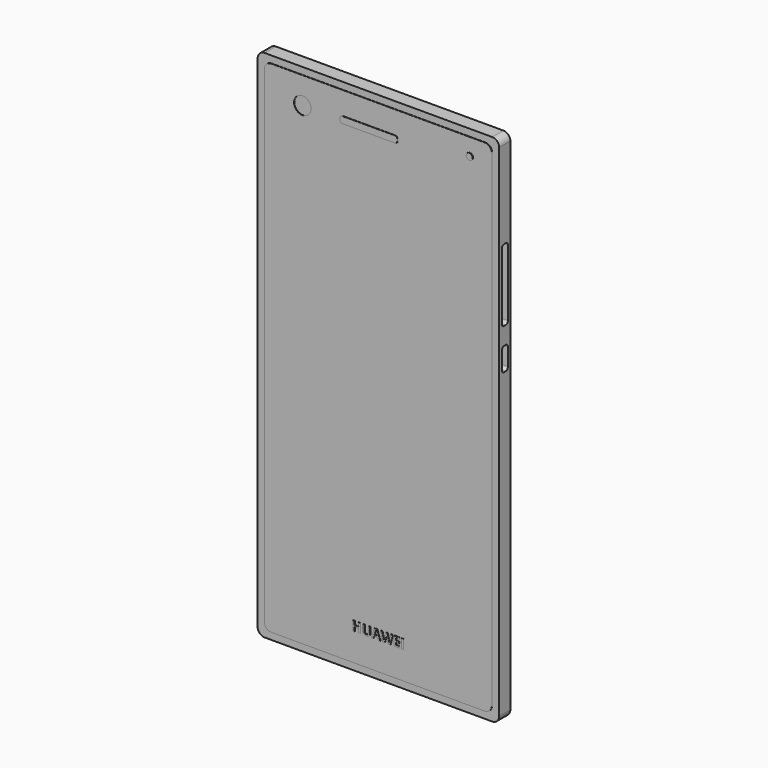
from build123d import *

# Parameters (mm, degrees)
F1_DEPTH      = 4
F3_DEPTH      = 2
F5_DEPTH      = 0.1
F6_W          = 64.8
F6_H          = 111
F7_DEPTH      = 0.1
F9_DEPTH      = 0.1
F10_R         = 2.4467451842
F11_DEPTH     = 0.1
F12_R         = 0.9273292915
F13_DEPTH     = 0.1
F14_TEXT_SIZE = 3.7091414883
F15_DEPTH     = 0.1


# Not quite as in the source:
# - Text() gives the source's letters only with a copy of the font that has no kerning and outlines rounded to 1/6400 em; it was checked with that copy


with BuildPart() as f1:
    # F0 (on Front) → F1 (new body)
    with BuildSketch(Plane.XZ):
        with BuildLine():
            ThreePointArc((-2, 0), (-0.5857864376, 0.5857864376), (0, 2))
            Line((0, 2), (0, 145))
            ThreePointArc((0, 145), (-0.5857864376, 146.4142135624), (-2, 147))
            Line((-2, 147), (-67, 147))
            ThreePointArc((-67, 147), (-68.4142135624, 146.4142135624), (-69, 145))
            Line((-69, 145), (-69, 2))
            ThreePointArc((-69, 2), (-68.4142135624, 0.5857864376), (-67, 0))
            Line((-67, 0), (-2, 0))
        make_face()
    extrude(amount=F1_DEPTH)

    # F2 (on face) → F3 (cut)
    with BuildSketch(Plane.YZ):
        with BuildLine():
            Line((-1.6547506675, 120), (-2.2547506675, 120))
            ThreePointArc((-2.2547506675, 120), (-2.8204360925, 119.7656854249), (-3.0547506675, 119.2))
            Line((-3.0547506675, 119.2), (-3.0547506675, 100.2))
            ThreePointArc((-3.0547506675, 100.2), (-2.8204360925, 99.6343145751), (-2.2547506675, 99.4))
            Line((-2.2547506675, 99.4), (-1.6547506675, 99.4))
            ThreePointArc((-1.6547506675, 99.4), (-1.0890652426, 99.6343145751), (-0.8547506675, 100.2))
            Line((-0.8547506675, 100.2), (-0.8547506675, 119.2))
            ThreePointArc((-0.8547506675, 119.2), (-1.0890652426, 119.7656854249), (-1.6547506675, 120))
        make_face()
        with BuildLine():
            Line((-1.6547506675, 94.4), (-2.2547506675, 94.4))
            ThreePointArc((-2.2547506675, 94.4), (-2.8204360925, 94.1656854249), (-3.0547506675, 93.6))
            Line((-3.0547506675, 93.6), (-3.0547506675, 88.6))
            ThreePointArc((-3.0547506675, 88.6), (-2.8204360925, 88.0343145751), (-2.2547506675, 87.8))
            Line((-2.2547506675, 87.8), (-1.6547506675, 87.8))
            ThreePointArc((-1.6547506675, 87.8), (-1.0890652426, 88.0343145751), (-0.8547506675, 88.6))
            Line((-0.8547506675, 88.6), (-0.8547506675, 93.6))
            ThreePointArc((-0.8547506675, 93.6), (-1.0890652426, 94.1656854249), (-1.6547506675, 94.4))
        make_face()
    extrude(amount=-F3_DEPTH, mode=Mode.SUBTRACT)

    # F6 (on face) → F7 (join)
    with BuildSketch(Plane.XZ.offset(4)):
        with Locations((-34.5, 75.5)):
            Rectangle(F6_W, F6_H)
    extrude(amount=F7_DEPTH)


with BuildPart() as f5:
    # F4 (on face) → F5 (new body)
    with BuildSketch(Plane.XZ.offset(4)):
        with BuildLine():
            Line((-4, 145), (-65, 145))
            ThreePointArc((-65, 145), (-66.4142135624, 144.4142135624), (-67, 143))
            Line((-67, 143), (-67, 4))
            ThreePointArc((-67, 4), (-66.4142135624, 2.5857864376), (-65, 2))
            Line((-65, 2), (-4, 2))
            ThreePointArc((-4, 2), (-2.5857864376, 2.5857864376), (-2, 4))
            Line((-2, 4), (-2, 143))
            ThreePointArc((-2, 143), (-2.5857864376, 144.4142135624), (-4, 145))
        make_face()
    extrude(amount=F5_DEPTH)

    # F10 (on face) → F11 (cut)
    with BuildSketch(Plane.XZ.offset(4.1)):
        with Locations((-56.0637563467, 137.3738348484)):
            Circle(F10_R)
    extrude(amount=-F11_DEPTH, mode=Mode.SUBTRACT)


with BuildPart() as f9:
    # F8 (on face) → F9 (new body)
    with BuildSketch(Plane.XZ.offset(4.1)):
        with BuildLine():
            Line((-29.6361570835, 138.4827951908), (-44.6361570835, 138.4827951908))
            ThreePointArc((-44.6361570835, 138.4827951908), (-45.1311318303, 138.2777699376), (-45.3361570835, 137.7827951908))
            Line((-45.3361570835, 137.7827951908), (-45.3361570835, 137.2827951908))
            ThreePointArc((-45.3361570835, 137.2827951908), (-45.1311318303, 136.787820444), (-44.6361570835, 136.5827951908))
            Line((-44.6361570835, 136.5827951908), (-29.6361570835, 136.5827951908))
            ThreePointArc((-29.6361570835, 136.5827951908), (-29.1411823367, 136.787820444), (-28.9361570835, 137.2827951908))
            Line((-28.9361570835, 137.2827951908), (-28.9361570835, 137.7827951908))
            ThreePointArc((-28.9361570835, 137.7827951908), (-29.1411823367, 138.2777699376), (-29.6361570835, 138.4827951908))
        make_face()
    extrude(amount=F9_DEPTH)


with BuildPart() as f13:
    # F12 (on face) → F13 (new body)
    with BuildSketch(Plane.XZ.offset(4.1)):
        with Locations((-8.3319898695, 140.1041597128)):
            Circle(F12_R)
    extrude(amount=F13_DEPTH)


with BuildPart() as f15:
    # F14 (on face) → F15 (new body)
    with BuildSketch(Plane.XZ.offset(4.1)):
        with Locations((-42, 10)):
            Text('HUAWEI', F14_TEXT_SIZE, font='Open Sans', font_style=FontStyle.BOLD, text_align=(TextAlign.LEFT, TextAlign.BOTTOM))
    extrude(amount=F15_DEPTH)


solid = Compound([f1.part, f5.part, f9.part, f13.part, f15.part])
